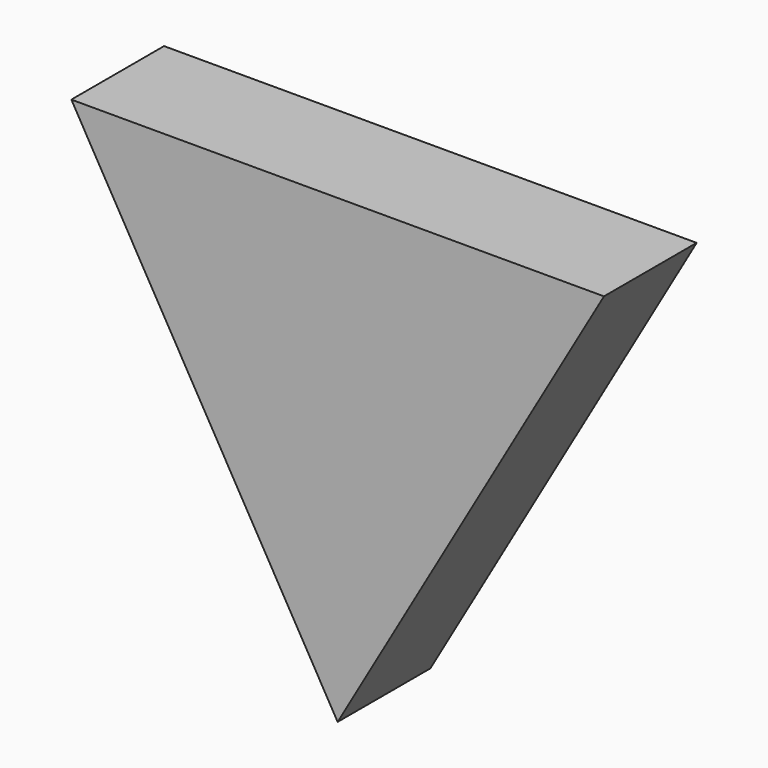
from build123d import *

# Parameters (mm, degrees)
F1_DEPTH = 25.4


# Not quite as in the source:
# - the program builds the solid bodies; features that only make, move or delete a surface that nothing else refers to are left out


with BuildPart() as f1:
    # F0 (on Front) → F1 (new body)
    with BuildSketch(Plane.XZ):
        Polygon((-58.3803272086, 33.7058976293), (0, -67.4117952585), (58.3803272086, 33.7058976293), align=None)
    extrude(amount=F1_DEPTH)


solid = f1.part
